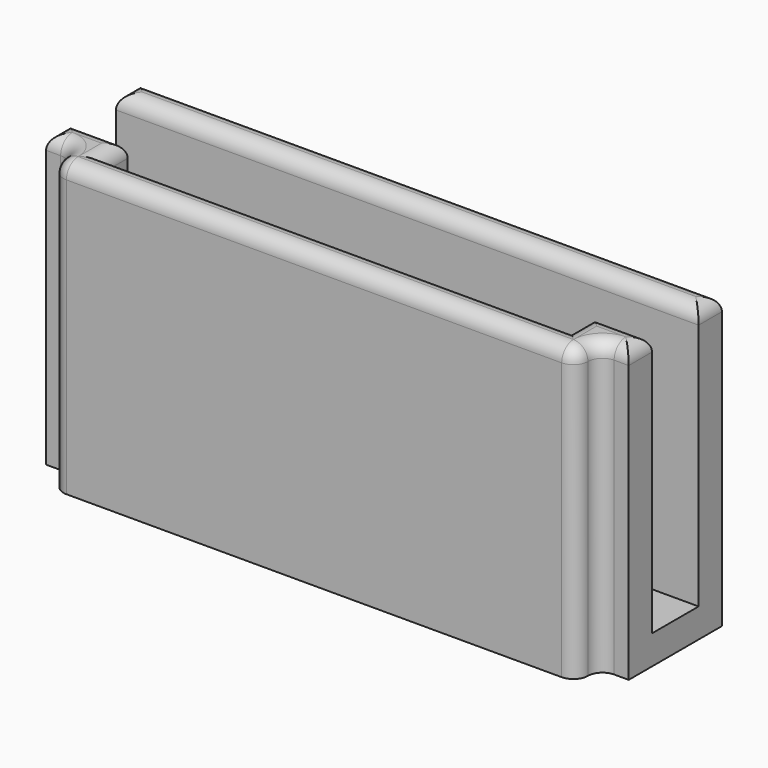
from build123d import *

# Parameters (mm, degrees)
F0_W     = 16
F0_H     = 1
F1_DEPTH = 1
F0_W_2   = 20
F2_DEPTH = 10
F3_R     = 0.49999


# Not quite as in the source:
# - a fillet or chamfer is up to 0.001 mm smaller than in the source, because OpenCascade refuses the exact size


with BuildPart() as f1:
    # F0 (on Top) → F1 (new body)
    with BuildSketch(Plane.XY):
        Polygon((10, 1), (-10, 1), (-10, -1), (-8, -1), (8, -1), (10, -1), align=None)
        with Locations((0, -1.5)):
            Rectangle(F0_W, F0_H)
    extrude(amount=F1_DEPTH)

    # F0 (on Top) → F2 (join)
    with BuildSketch(Plane.XY):
        with Locations((0, 1.5)):
            Rectangle(F0_W_2, F0_H)
        Polygon((-8, -1), (-10, -1), (-10, -2), (-9, -2), (-8, -2), align=None)
        Polygon((8, -2), (-8, -2), (-9, -2), (-9, -3), (9, -3), (9, -2), align=None)
        Polygon((10, -2), (10, -1), (8, -1), (8, -2), (9, -2), align=None)
    extrude(amount=F2_DEPTH)

    # F3 (radius 0.5 in the source; OpenCascade refuses exactly that, so slightly less here)
    f3_edges = [f1.edges().sort_by_distance(p)[0] for p in [
        (-9, -2, 5),
        (-9, -3, 5),
        (9, -2, 5),
        (9, -3, 5),
        (-9, -1, 10),
        (-10, -1.5, 10),
        (-9.5, -2, 10),
        (-9, -2.5, 10),
        (0, -3, 10),
        (9, -2.5, 10),
        (9.5, -2, 10),
        (10, -1.5, 10),
        (9, -1, 10),
        (8, -1.5, 10),
        (0, -2, 10),
        (-8, -1.5, 10),
        (-10, 1.5, 10),
        (0, 1, 10),
        (10, 1.5, 10),
        (0, 2, 10),
    ]]
    fillet(f3_edges, radius=F3_R)


solid = f1.part
